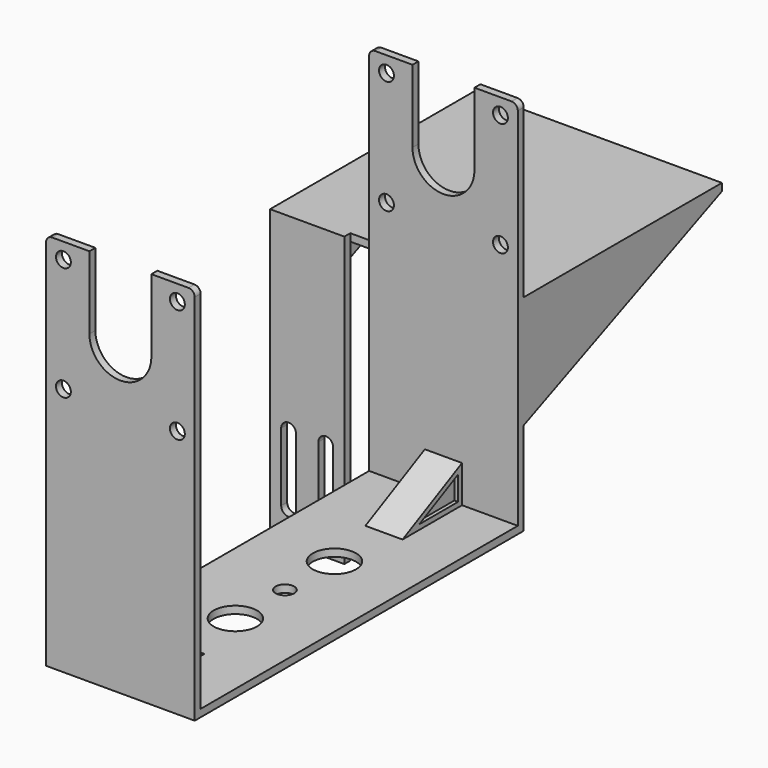
from build123d import *

# Parameters (mm, degrees)
F2_W      = 120
F2_H      = 6
F5_D      = 12
F7_DEPTH  = 332
F9_DEPTH  = 15
F11_DEPTH = 3
F12_R     = 5
F14_D     = 35
F15_D     = 15
F16_W     = 200
F16_H     = 6
F17_DEPTH = 200
F18_DEPTH = 6
F19_W     = 60
F19_H     = 6
F19_H_2   = 226.75
F20_DEPTH = 6
F22_DEPTH = 6


# Not quite as in the source:
# - a pattern or mirror of a feature is missing from the dataset's text; its kind, count and spacing are read off the source's solid


with BuildPart() as f3:
    # F3: sweep along a path in F0
    with BuildLine(Plane.YZ) as f3_path:
        Line((-160, 150), (-160, -150))
        Line((-160, -150), (160, -150))
        Line((160, -150), (160, 150))
    # F2 (on offset) → F3 (sweep)
    with BuildSketch(Plane.XY.offset(150)):
        with Locations((0, -163)):
            Rectangle(F2_W, F2_H)
    sweep(path=f3_path.line, transition=Transition.RIGHT)

    # F5 (through all)
    with Locations(Plane.XZ.offset(166)):
        with Locations((-46, 137.25), (-46, 45.25), (46, 45.25), (46, 137.25)):
            Hole(F5_D / 2)

    # F6 (on face) → F7 (cut, through all)
    with BuildSketch(Plane.XZ.offset(166)):
        with BuildLine():
            Line((25, 150), (-25, 150))
            Line((-25, 150), (-25, 91.25))
            ThreePointArc((-25, 91.25), (0, 66.25), (25, 91.25))
            Line((25, 91.25), (25, 150))
        make_face()
    extrude(amount=-F7_DEPTH, mode=Mode.SUBTRACT)

    # F8 (on Right) → F9 (join, symmetric)
    with BuildSketch(Plane.YZ):
        Polygon((160, -150), (160, -120), (100, -150), align=None)
    f9 = extrude(amount=F9_DEPTH, both=True)

    # F9_copies: F9 across plane
    add(f9.mirror(Plane(origin=(0, 0, 0), x_dir=(0, 0, -1), z_dir=(0, -1, 0))))

    # F10 (on face) → F11 (cut)
    with BuildSketch(Plane.YZ.offset(15)):
        Polygon((116.94427191, -146), (156, -146), (156, -126.472135955), align=None)
    f11 = extrude(amount=-F11_DEPTH, mode=Mode.SUBTRACT)

    # F11_copies: F11 across plane
    add(f11.mirror(Plane(origin=(0, 0, 0), x_dir=(0, 0, -1), z_dir=(-1, 0, 0))), mode=Mode.SUBTRACT)

    # F11_copies1: F11 across plane
    add(f11.mirror(Plane(origin=(0, 0, 0), x_dir=(0, 0, -1), z_dir=(0, -1, 0))), mode=Mode.SUBTRACT)

    # F12
    f12_edges = [f3.edges().sort_by_distance(p)[0] for p in [
        (60, -163, 150),
        (-60, -163, 150),
        (-60, 163, 150),
        (60, 163, 150),
    ]]
    fillet(f12_edges, radius=F12_R)

    # F14 (through all)
    with Locations(Plane.XY.offset(-150)):
        with Locations((0, 50), (0, -50)):
            Hole(F14_D / 2)

    # F15 (through all)
    with Locations(Plane.XY.offset(-150)):
        with Locations((0, 0)):
            Hole(F15_D / 2)

    # F16 (on face) → F17 (join)
    with BuildSketch(Plane.YZ.offset(60)):
        with Locations((266, 7)):
            Rectangle(F16_W, F16_H)
    extrude(amount=-F17_DEPTH)

    # F16 (on face) → F18 (join)
    with BuildSketch(Plane.YZ.offset(60)):
        Polygon((366, 4), (166, 4), (166, -81), align=None)
    f18 = extrude(amount=-F18_DEPTH)

    # F18_copies: F18 across plane
    add(f18.mirror(Plane(origin=(0, 0, 0), x_dir=(0, 0, -1), z_dir=(-1, 0, 0))))

    # F19 (on face) → F20 (join)
    with BuildSketch(Plane.XZ.offset(-166)):
        with Locations((-110, 7)):
            Rectangle(F19_W, F19_H)
        with Locations((-110, -109.375)):
            Rectangle(F19_W, F19_H_2)
        with BuildLine():
            ThreePointArc((-131, -142.75), (-125, -136.75), (-119, -142.75))
            Line((-119, -142.75), (-119, -197.75))
            ThreePointArc((-119, -197.75), (-125, -203.75), (-131, -197.75))
            Line((-131, -197.75), (-131, -142.75))
        make_face(mode=Mode.SUBTRACT)
        with BuildLine():
            Line((-101, -197.75), (-101, -142.75))
            ThreePointArc((-101, -142.75), (-95, -136.75), (-89, -142.75))
            Line((-89, -142.75), (-89, -197.75))
            ThreePointArc((-89, -197.75), (-95, -203.75), (-101, -197.75))
        make_face(mode=Mode.SUBTRACT)
    extrude(amount=F20_DEPTH)

    # F21 (on face) → F22 (join)
    with BuildSketch(Plane(origin=(-140, 0, 0), x_dir=(0, -1, 0), z_dir=(-1, 0, 0))):
        Polygon((-166, -81), (-166, 4), (-366, 4), align=None)
    extrude(amount=-F22_DEPTH)


solid = f3.part
